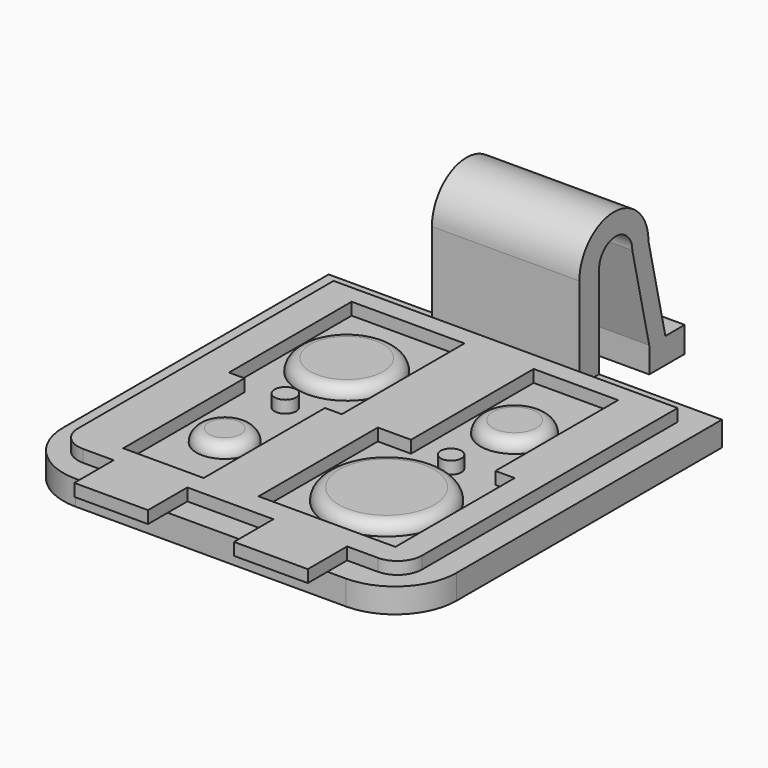
from build123d import *

# Parameters (mm, degrees)
F0_W      = 32
F0_H      = 32
F1_DEPTH  = 2
F2_W      = 6
F2_H      = 2
F3_DEPTH  = 1
F4_R      = 5
F5_R      = 2
F6_R      = 5
F6_R_2    = 4.75
F7_DEPTH  = 0.5
F6_R_3    = 4.5
F8_DEPTH  = 1
F9_R      = 0.1
F10_R     = 0.1
F11_W     = 6.8694591671
F11_H     = 12.4790910631
F12_DEPTH = 1
F13_R     = 3.9747540769
F13_R_2   = 0.8810664351
F13_R_3   = 2.2905042987
F14_DEPTH = 1
F15_R     = 0.99999
F16_R     = 2.7689113732
F16_R_2   = 0.8414057699
F16_R_3   = 4.8736093879
F17_DEPTH = 1
F18_R     = 0.99999
F20_W     = 2
F20_H     = 7.5
F21_DEPTH = 12


# Not quite as in the source:
# - a fillet or chamfer is up to 0.001 mm smaller than in the source, because OpenCascade refuses the exact size


with BuildPart() as f1:
    # F0 (on Top) → F1 (new body)
    with BuildSketch(Plane.XY):
        Rectangle(F0_W, F0_H)
    extrude(amount=-F1_DEPTH)

    # F2 (on face) → F3 (join)
    with BuildSketch(Plane.XY):
        Polygon((14, 14), (-14, 14), (-14, -14), (-9.5, -14), (-3.5, -14), (3.5, -14), (9.5, -14), (14, -14), align=None)
        with Locations((6.5, -17)):
            Rectangle(F2_W, F2_H)
        with Locations((6.5, -15)):
            Rectangle(F2_W, F2_H)
        with Locations((-6.5, -17)):
            Rectangle(F2_W, F2_H)
        with Locations((-6.5, -15)):
            Rectangle(F2_W, F2_H)
    extrude(amount=F3_DEPTH)

    # F4
    f4_edges = [f1.edges().sort_by_distance(p)[0] for p in [
        (-16, -16, -1),
        (16, -16, -1),
    ]]
    fillet(f4_edges, radius=F4_R)

    # F5
    f5_edges = [f1.edges().sort_by_distance(p)[0] for p in [
        (-14, -14, 0.5),
        (14, -14, 0.5),
    ]]
    fillet(f5_edges, radius=F5_R)

    # F6 (on face) → F7 (join)
    with BuildSketch(Plane(origin=(0, 0, -2), x_dir=(1, 0, 0), z_dir=(0, 0, -1))):
        with Locations((-7.96, 10)):
            Circle(F6_R)
        with Locations((-7.96, 10)):
            Circle(F6_R_2, mode=Mode.SUBTRACT)
        with BuildLine():
            ThreePointArc((12.9630157733, 10), (7.9630157733, 15), (2.9630157733, 10))
            ThreePointArc((2.9630157733, 10), (7.9630157733, 5), (12.9630157733, 10))
        make_face()
        with BuildLine():
            ThreePointArc((12.7130157733, 10), (7.9630157733, 5.25), (3.2130157733, 10))
            ThreePointArc((3.2130157733, 10), (7.9630157733, 14.75), (12.7130157733, 10))
        make_face(mode=Mode.SUBTRACT)
    extrude(amount=F7_DEPTH)

    # F6 (on face) → F8 (join)
    with BuildSketch(Plane(origin=(0, 0, -2), x_dir=(1, 0, 0), z_dir=(0, 0, -1))):
        with Locations((-7.96, 10)):
            Circle(F6_R_3)
        with BuildLine():
            ThreePointArc((12.4630157733, 10), (7.9630157733, 14.5), (3.4630157733, 10))
            ThreePointArc((3.4630157733, 10), (7.9630157733, 5.5), (12.4630157733, 10))
        make_face()
    extrude(amount=F8_DEPTH)

    # F9
    f9_edges = [f1.edges().sort_by_distance(p)[0] for p in [
        (-12.96, -10, -2.5),
    ]]
    fillet(f9_edges, radius=F9_R)

    # F10
    f10_edges = [f1.edges().sort_by_distance(p)[0] for p in [
        (12.963016, -10, -2.5),
    ]]
    fillet(f10_edges, radius=F10_R)

    # F11 (on face) → F12 (cut)
    with BuildSketch(Plane.XY.offset(1)):
        Polygon((-10.0488252938, -12.3401368037), (-3.5, -12.3401368037), (-3.5, 0), (-7.3588341475, 0), (-10.0488252938, 0), align=None)
        Polygon((-7.3588341475, 0), (-3.5, 0), (-2.1322800312, 0), (-2.1322800312, 12.4790910631), (-11.3117620349, 12.4790910631), (-11.3117620349, 0), (-10.0488252938, 0), align=None)
        with Locations((6.9347295836, 6.2395455316)):
            Rectangle(F11_W, F11_H)
        Polygon((0.7984698168, 0), (0.7984698168, -12.129846029), (11.932070367, -12.129846029), (11.932070367, 0), (10.3694591671, 0), (3.5, 0), align=None)
    extrude(amount=-F12_DEPTH, mode=Mode.SUBTRACT)

    # F13 (on face) → F14 (join)
    with BuildSketch(Plane.XY):
        with Locations((-6.7220210331, 6.2395455316)):
            Circle(F13_R)
        with Locations((-6.7220210331, 0)):
            Circle(F13_R_2)
        with Locations((-6.7220210331, -6.1700684018)):
            Circle(F13_R_3)
    extrude(amount=F14_DEPTH)

    # F15 (radius 1 in the source; OpenCascade refuses exactly that, so slightly less here)
    f15_edges = [f1.edges().sort_by_distance(p)[0] for p in [
        (-10.696775, 6.239546, 1),
        (-9.012525, -6.170068, 1),
    ]]
    fillet(f15_edges, radius=F15_R)

    # F16 (on face) → F17 (join)
    with BuildSketch(Plane.XY):
        with Locations((6.9347295836, 6.2395455316)):
            Circle(F16_R)
        with Locations((6.7594647408, 0)):
            Circle(F16_R_2)
        with Locations((6.3652700919, -6.0649230145)):
            Circle(F16_R_3)
    extrude(amount=F17_DEPTH)

    # F18 (radius 1 in the source; OpenCascade refuses exactly that, so slightly less here)
    f18_edges = [f1.edges().sort_by_distance(p)[0] for p in [
        (4.165818, 6.239546, 1),
        (1.491661, -6.064923, 1),
    ]]
    fillet(f18_edges, radius=F18_R)

    # F20 (on offset) → F21 (join)
    with BuildSketch(Plane.YZ.offset(6)):
        with Locations((15, 3.75)):
            Rectangle(F20_W, F20_H)
        with BuildLine():
            ThreePointArc((21.0264474154, 7.5), (17.5132237077, 11.0132237077), (14, 7.5))
            Line((14, 7.5), (16, 7.5))
            ThreePointArc((16, 7.5), (17.6929781139, 9.1929781139), (19.3859562278, 7.5))
            Line((19.3859562278, 7.5), (21.1084708571, 0))
            Line((21.1084708571, 0), (22.7489620447, 0))
            Line((22.7489620447, 0), (21.0264474154, 7.5))
        make_face()
        Polygon((24.7175507247, 0), (22.7489620447, 0), (21.1084708571, 0), (21.1084708571, -2.0891015884), (24.7175507247, -2.0891015884), align=None)
    extrude(amount=-F21_DEPTH)


solid = f1.part
